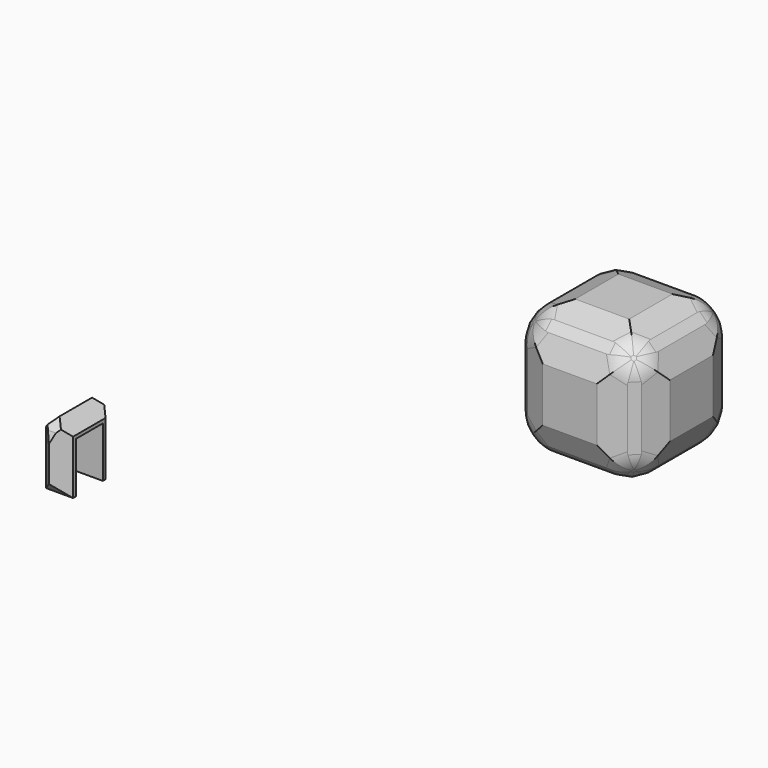
from build123d import *

# Parameters (mm, degrees)
F0_W         = 25.4
F0_H         = 25.4
F1_DEPTH     = 25.4
F2_SIZE      = 5.08
F3_C1_SIZE   = 2.54
F3_C2_SIZE   = 2.54
F3_C3_SIZE   = 2.54
F3_C4_SIZE   = 2.54
F3_C5_SIZE   = 2.54
F3_C6_SIZE   = 2.54
F3_C7_SIZE   = 2.54
F3_C8_SIZE   = 2.54
F3_C9_SIZE   = 2.54
F3_C10_SIZE  = 2.54
F3_C11_SIZE  = 2.54
F3_C12_SIZE  = 2.54
F3_C13_SIZE  = 2.54
F3_C14_SIZE  = 2.54
F3_C15_SIZE  = 2.54
F3_C16_SIZE  = 2.54
F3_C17_SIZE  = 2.54
F3_C18_SIZE  = 2.54
F3_C19_SIZE  = 2.54
F3_C20_SIZE  = 2.54
F3_C21_SIZE  = 2.54
F3_C22_SIZE  = 2.54
F3_C23_SIZE  = 2.54
F3_C24_SIZE  = 2.54
F4_R         = 5.08
F5_W         = 5.08
F5_H         = 12.7
F6_DEPTH     = 12.7
F7_W         = 6.35
F7_H         = 9.525
F8_DEPTH     = 5.08
F9_SIZE      = 2.53999
F10_T1_DEPTH = 23.2241595789
F10_T3_DEPTH = 10.8131399699
F10_T5_DEPTH = 18.1441495789


# Not quite as in the source:
# - a fillet or chamfer that OpenCascade refuses, or shapes differently, is made with other operations: its cross-section is extruded or revolved along the edge and cut away or added
# - a fillet or chamfer is up to 0.001 mm smaller than in the source, because OpenCascade refuses the exact size


with BuildPart() as f1:
    # F0 (on Top) → F1 (new body)
    with BuildSketch(Plane.XY):
        with Locations((12.7, 11.1038634095)):
            Rectangle(F0_W, F0_H)
    extrude(amount=F1_DEPTH)

    # F2
    f2_edges = [f1.edges().sort_by_distance(p)[0] for p in [
        (12.7, 23.803863, 25.4),
        (0, 11.103863, 25.4),
        (12.7, -1.596137, 25.4),
        (25.4, 11.103863, 25.4),
        (25.4, -1.596137, 12.7),
        (25.4, 23.803863, 12.7),
        (25.4, 11.103863, 0),
        (0, -1.596137, 12.7),
        (12.7, -1.596137, 0),
        (0, 23.803863, 12.7),
        (0, 11.103863, 0),
        (12.7, 23.803863, 0),
    ]]
    chamfer(f2_edges, length=F2_SIZE)

    # F3: chamfer of 2.54 on 24 edges, made by hand

    # F3_c1
    f3_c1_edges = [f1.edges().sort_by_distance(p)[0] for p in [
        (12.7, 23.8038634095, 20.32),
    ]]
    chamfer(f3_c1_edges, length=F3_C1_SIZE)

    # F3_c2
    f3_c2_edges = [f1.edges().sort_by_distance(p)[0] for p in [
        (20.32, 23.8038634095, 11.43),
    ]]
    chamfer(f3_c2_edges, length=F3_C2_SIZE)

    # F3_c3
    f3_c3_edges = [f1.edges().sort_by_distance(p)[0] for p in [
        (5.08, 23.8038634095, 11.43),
    ]]
    chamfer(f3_c3_edges, length=F3_C3_SIZE)

    # F3_c4
    f3_c4_edges = [f1.edges().sort_by_distance(p)[0] for p in [
        (12.7, 23.8038634095, 5.08),
    ]]
    chamfer(f3_c4_edges, length=F3_C4_SIZE)

    # F3_c5
    f3_c5_edges = [f1.edges().sort_by_distance(p)[0] for p in [
        (12.7, 18.7238634095, 25.4),
    ]]
    chamfer(f3_c5_edges, length=F3_C5_SIZE)

    # F3_c6
    f3_c6_edges = [f1.edges().sort_by_distance(p)[0] for p in [
        (25.4, 18.7238634095, 12.7),
    ]]
    chamfer(f3_c6_edges, length=F3_C6_SIZE)

    # F3_c7
    f3_c7_edges = [f1.edges().sort_by_distance(p)[0] for p in [
        (0, 18.7238634095, 12.7),
    ]]
    chamfer(f3_c7_edges, length=F3_C7_SIZE)

    # F3_c8
    f3_c8_edges = [f1.edges().sort_by_distance(p)[0] for p in [
        (12.7, 18.7238634095, 0),
    ]]
    chamfer(f3_c8_edges, length=F3_C8_SIZE)

    # F3_c9
    f3_c9_edges = [f1.edges().sort_by_distance(p)[0] for p in [
        (20.32, 9.8338634095, 25.4),
    ]]
    chamfer(f3_c9_edges, length=F3_C9_SIZE)

    # F3_c10
    f3_c10_edges = [f1.edges().sort_by_distance(p)[0] for p in [
        (5.08, 9.8338634095, 25.4),
    ]]
    chamfer(f3_c10_edges, length=F3_C10_SIZE)

    # F3_c11
    f3_c11_edges = [f1.edges().sort_by_distance(p)[0] for p in [
        (12.7, 3.4838634095, 25.4),
    ]]
    chamfer(f3_c11_edges, length=F3_C11_SIZE)

    # F3_c12
    f3_c12_edges = [f1.edges().sort_by_distance(p)[0] for p in [
        (25.4, 9.8338634095, 20.32),
    ]]
    chamfer(f3_c12_edges, length=F3_C12_SIZE)

    # F3_c13
    f3_c13_edges = [f1.edges().sort_by_distance(p)[0] for p in [
        (25.4, 3.4838634095, 11.43),
    ]]
    chamfer(f3_c13_edges, length=F3_C13_SIZE)

    # F3_c14
    f3_c14_edges = [f1.edges().sort_by_distance(p)[0] for p in [
        (25.4, 11.1038634095, 5.08),
    ]]
    chamfer(f3_c14_edges, length=F3_C14_SIZE)

    # F3_c15
    f3_c15_edges = [f1.edges().sort_by_distance(p)[0] for p in [
        (0, 9.8338634095, 20.32),
    ]]
    chamfer(f3_c15_edges, length=F3_C15_SIZE)

    # F3_c16
    f3_c16_edges = [f1.edges().sort_by_distance(p)[0] for p in [
        (0, 3.4838634095, 11.43),
    ]]
    chamfer(f3_c16_edges, length=F3_C16_SIZE)

    # F3_c17
    f3_c17_edges = [f1.edges().sort_by_distance(p)[0] for p in [
        (0, 11.1038634095, 5.08),
    ]]
    chamfer(f3_c17_edges, length=F3_C17_SIZE)

    # F3_c18
    f3_c18_edges = [f1.edges().sort_by_distance(p)[0] for p in [
        (20.32, 9.8338634095, 0),
    ]]
    chamfer(f3_c18_edges, length=F3_C18_SIZE)

    # F3_c19
    f3_c19_edges = [f1.edges().sort_by_distance(p)[0] for p in [
        (11.43, 3.4838634095, 0),
    ]]
    chamfer(f3_c19_edges, length=F3_C19_SIZE)

    # F3_c20
    f3_c20_edges = [f1.edges().sort_by_distance(p)[0] for p in [
        (5.08, 11.1038634095, 0),
    ]]
    chamfer(f3_c20_edges, length=F3_C20_SIZE)

    # F3_c21
    f3_c21_edges = [f1.edges().sort_by_distance(p)[0] for p in [
        (12.7, -1.5961365905, 20.32),
    ]]
    chamfer(f3_c21_edges, length=F3_C21_SIZE)

    # F3_c22
    f3_c22_edges = [f1.edges().sort_by_distance(p)[0] for p in [
        (20.32, -1.5961365905, 11.43),
    ]]
    chamfer(f3_c22_edges, length=F3_C22_SIZE)

    # F3_c23
    f3_c23_edges = [f1.edges().sort_by_distance(p)[0] for p in [
        (5.08, -1.5961365905, 11.43),
    ]]
    chamfer(f3_c23_edges, length=F3_C23_SIZE)

    # F3_c24
    f3_c24_edges = [f1.edges().sort_by_distance(p)[0] for p in [
        (12.7, -1.5961365905, 5.08),
    ]]
    chamfer(f3_c24_edges, length=F3_C24_SIZE)

    # F4
    f4_edges = [f1.edges().sort_by_distance(p)[0] for p in [
        (2.54, 21.263863, 5.08),
        (2.54, 21.263863, 20.32),
        (2.54, 0.943863, 5.08),
        (2.54, 0.943863, 20.32),
        (22.86, 0.943863, 20.32),
        (22.86, 0.943863, 5.08),
        (22.86, 21.263863, 5.08),
        (22.86, 21.263863, 20.32),
        (3.850245, -0.034653, 4.748271),
        (3.850245, -0.034653, 20.651729),
        (4.748271, -0.034653, 3.850245),
        (20.651729, -0.034653, 3.850245),
        (4.748271, -0.034653, 21.549755),
        (20.651729, -0.034653, 21.549755),
        (21.549755, -0.034653, 4.748271),
        (21.549755, -0.034653, 20.651729),
        (5.08, 0.943863, 2.54),
        (4.748271, 2.254109, 1.561483),
        (3.850245, 3.152134, 1.561483),
        (2.54, 3.483863, 2.54),
        (1.561483, 2.254109, 4.748271),
        (1.561483, 3.152134, 3.850245),
        (1.561483, 2.254109, 20.651729),
        (1.561483, 3.152134, 21.549755),
        (5.08, 0.943863, 22.86),
        (2.54, 3.483863, 22.86),
        (4.748271, 2.254109, 23.838517),
        (3.850245, 3.152134, 23.838517),
        (20.32, 0.943863, 2.54),
        (20.651729, 2.254109, 1.561483),
        (21.549755, 3.152134, 1.561483),
        (22.86, 3.483863, 2.54),
        (23.838517, 2.254109, 4.748271),
        (23.838517, 3.152134, 3.850245),
        (23.838517, 2.254109, 20.651729),
        (23.838517, 3.152134, 21.549755),
        (20.32, 0.943863, 22.86),
        (22.86, 3.483863, 22.86),
        (20.651729, 2.254109, 23.838517),
        (21.549755, 3.152134, 23.838517),
        (3.850245, 19.055592, 1.561483),
        (2.54, 18.723863, 2.54),
        (1.561483, 19.055592, 3.850245),
        (1.561483, 19.055592, 21.549755),
        (2.54, 18.723863, 22.86),
        (3.850245, 19.055592, 23.838517),
        (21.549755, 19.055592, 1.561483),
        (22.86, 18.723863, 2.54),
        (23.838517, 19.055592, 3.850245),
        (23.838517, 19.055592, 21.549755),
        (22.86, 18.723863, 22.86),
        (21.549755, 19.055592, 23.838517),
        (4.748271, 19.953618, 1.561483),
        (1.561483, 19.953618, 4.748271),
        (5.08, 21.263863, 2.54),
        (4.748271, 22.24238, 3.850245),
        (3.850245, 22.24238, 4.748271),
        (20.651729, 19.953618, 1.561483),
        (1.561483, 19.953618, 20.651729),
        (4.748271, 19.953618, 23.838517),
        (5.08, 21.263863, 22.86),
        (3.850245, 22.24238, 20.651729),
        (4.748271, 22.24238, 21.549755),
        (20.651729, 19.953618, 23.838517),
        (23.838517, 19.953618, 4.748271),
        (20.32, 21.263863, 2.54),
        (20.651729, 22.24238, 3.850245),
        (21.549755, 22.24238, 4.748271),
        (23.838517, 19.953618, 20.651729),
        (20.32, 21.263863, 22.86),
        (21.549755, 22.24238, 20.651729),
        (20.651729, 22.24238, 21.549755),
    ]]
    fillet(f4_edges, radius=F4_R)


with BuildPart() as f6:
    # F5 (on Top) → F6 (new body)
    with BuildSketch(Plane.XY):
        with Locations((-43.4196100876, -47.4590435624)):
            Rectangle(F5_W, F5_H)
    extrude(amount=F6_DEPTH)

    # F7 (on face) → F8 (cut)
    with BuildSketch(Plane.YZ.offset(-40.8796100876)):
        with Locations((-47.4590435624, 4.7625)):
            Rectangle(F7_W, F7_H)
    extrude(amount=-F8_DEPTH, mode=Mode.SUBTRACT)

    # F9 (size 2.54 in the source; OpenCascade refuses exactly that, so slightly less here)
    f9_edges = [f6.edges().sort_by_distance(p)[0] for p in [
        (-43.41961, -41.109044, 12.7),
        (-45.95961, -47.459044, 12.7),
        (-43.41961, -53.809044, 12.7),
        (-40.87961, -47.459044, 12.7),
    ]]
    chamfer(f9_edges, length=F9_SIZE)

    # F10: chamfer of 2.54 on 8 edges, made by hand

    # F10_s2 → F10_t1 (cut)
    with BuildSketch(Plane.XY.offset(-6.5320747894)):
        Polygon((-45.9596100876, -51.2690435624), (-43.4196100876, -53.8090435624), (-45.9596100876, -53.8090435624), align=None)
        Polygon((-40.8796100876, -51.2690435624), (-43.4196100876, -53.8090435624), (-40.8796100876, -53.8090435624), align=None)
        Polygon((-43.4196100876, -41.1090435624), (-40.8796100876, -43.6490435624), (-40.8796100876, -41.1090435624), align=None)
        Polygon((-43.4196100876, -41.1090435624), (-45.9596100876, -43.6490435624), (-45.9596100876, -41.1090435624), align=None)
    extrude(amount=F10_T1_DEPTH, mode=Mode.SUBTRACT)

    # F10_s4 → F10_t3 (cut)
    with BuildSketch(Plane.YZ.offset(-48.8261800726)):
        Polygon((-53.8090435624, 9.1079075516), (-53.0650947866, 10.9039587758), (-53.8090435624, 10.16001), align=None)
        Polygon((-41.1090435624, 9.1079075516), (-41.8529923382, 10.9039587758), (-41.1090435624, 10.16001), align=None)
    extrude(amount=F10_T3_DEPTH, mode=Mode.SUBTRACT)

    # F10_s6 → F10_t5 (cut)
    with BuildSketch(Plane.YZ.offset(-52.4916848771)):
        Polygon((-53.8090435624, 2.54), (-51.2690435624, 0), (-53.8090435624, 0), align=None)
        Polygon((-41.1090435624, 2.54), (-43.6490435624, 0), (-41.1090435624, 0), align=None)
    extrude(amount=F10_T5_DEPTH, mode=Mode.SUBTRACT)


solid = Compound([f1.part, f6.part])
